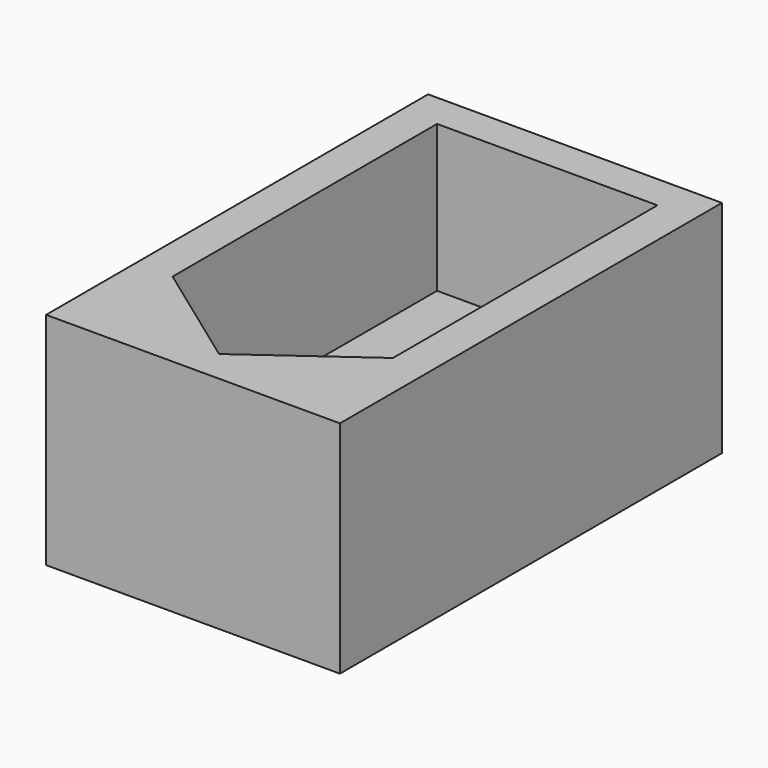
from build123d import *

# Parameters (mm, degrees)
F0_W     = 101.6
F0_H     = 165.1
F1_DEPTH = 76.2
F3_DEPTH = 50.8


# Not quite as in the source:
# - a feature names something its author has since deleted; it is built from what else it names


with BuildPart() as f1:
    # F0 (on Top) → F1 (new body)
    with BuildSketch(Plane.XY):
        with Locations((50.8, 82.55)):
            Rectangle(F0_W, F0_H)
    extrude(amount=F1_DEPTH)

    # F2 (on face) → F3 (cut)
    with BuildSketch(Plane.XY.offset(76.2)):
        Polygon((12.7, 38.8), (50.8, 11.2792805327), (88.9, 38.8), (88.9, 153.1), (50.8, 153.1), (12.7, 153.1), align=None)
    extrude(amount=-F3_DEPTH, mode=Mode.SUBTRACT)


solid = f1.part
